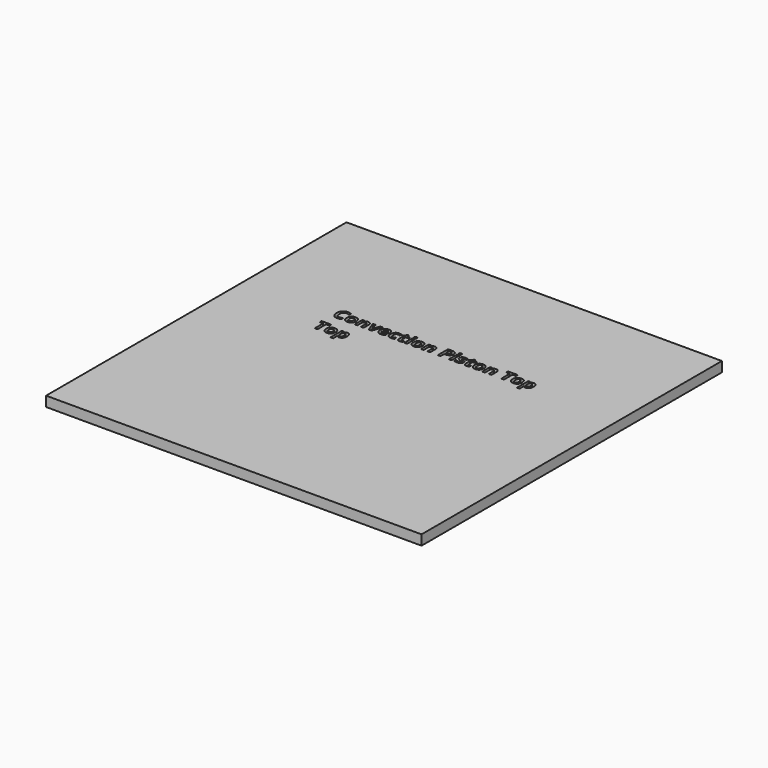
from build123d import *

# Parameters (mm, degrees)
F0_W         = 75
F0_H         = 75
F1_DEPTH     = 2
F2_TEXT_SIZE = 3.598892216
F3_DEPTH     = 25


# Not quite as in the source:
# - Text() gives the source's letters only with a copy of the font that has no kerning and outlines rounded to 1/6400 em; it was checked with that copy


with BuildPart() as f1:
    # F0 (on Top) → F1 (new body)
    with BuildSketch(Plane.XY):
        with Locations((-6.0041248798, 4.1450588199)):
            Rectangle(F0_W, F0_H)
    extrude(amount=F1_DEPTH)

    # F2 (on face) → F3 (cut)
    with BuildSketch(Plane.XY.offset(2)):
        with Locations((-25.7669769648, 15.4893149027)):
            Text('Convection Piston Top', F2_TEXT_SIZE, font='Open Sans', font_style=FontStyle.BOLD, text_align=(TextAlign.LEFT, TextAlign.BOTTOM))
        with Locations((-25.7669769648, 10.5948214889)):
            Text('Top', F2_TEXT_SIZE, font='Open Sans', font_style=FontStyle.BOLD, text_align=(TextAlign.LEFT, TextAlign.BOTTOM))
    extrude(amount=-F3_DEPTH, mode=Mode.SUBTRACT)


solid = f1.part
